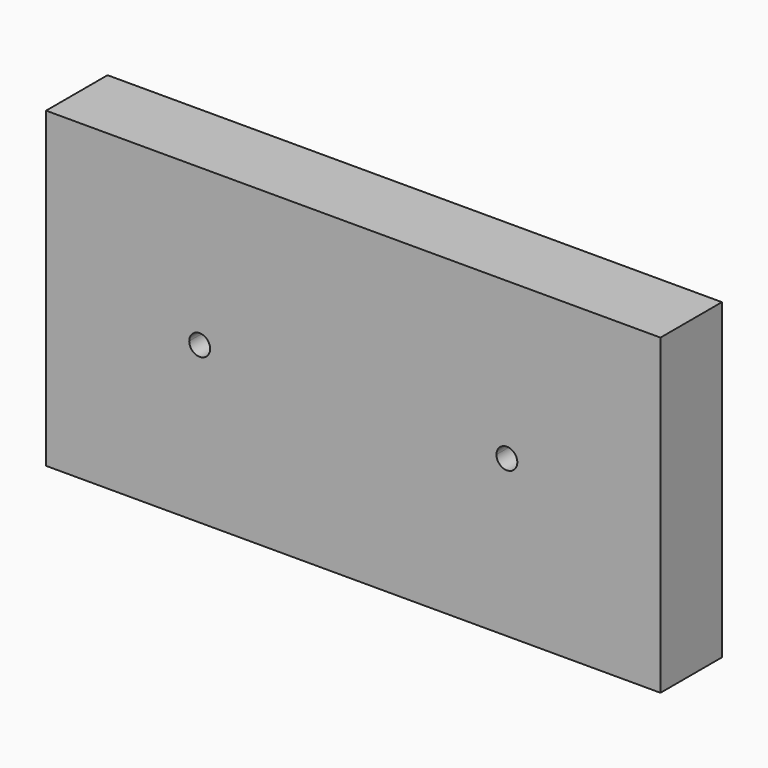
from build123d import *

# Parameters (mm, degrees)
F1_DEPTH = 3.175


with BuildPart() as f1:
    # F0 (on Front) → F1 (new body)
    with BuildSketch(Plane.XZ):
        with BuildLine():
            Line((-18.7849326355, 12.9286), (-25.1349326355, 12.9286))
            Line((-25.1349326355, 12.9286), (-25.1349326355, 6.4643))
            Line((-25.1349326355, 6.4643), (-19.2167326355, 6.4643))
            ThreePointArc((-19.2167326355, 6.4643), (-19.0902613436, 6.7696287081), (-18.7849326355, 6.8961))
            Line((-18.7849326355, 6.8961), (-18.7849326355, 12.9286))
        make_face()
        with BuildLine():
            Line((-12.4349326355, 12.9286), (-18.7849326355, 12.9286))
            Line((-18.7849326355, 12.9286), (-18.7849326355, 6.8961))
            ThreePointArc((-18.7849326355, 6.8961), (-18.4796039274, 6.7696287081), (-18.3531326355, 6.4643))
            Line((-18.3531326355, 6.4643), (-12.4349326355, 6.4643))
            Line((-12.4349326355, 6.4643), (-12.4349326355, 12.9286))
        make_face()
        with BuildLine():
            Line((-6.0849326355, 12.9286), (-12.4349326355, 12.9286))
            Line((-12.4349326355, 12.9286), (-12.4349326355, 6.4643))
            Line((-12.4349326355, 6.4643), (-6.5167326355, 6.4643))
            ThreePointArc((-6.5167326355, 6.4643), (-6.3902613436, 6.7696287081), (-6.0849326355, 6.8961))
            Line((-6.0849326355, 6.8961), (-6.0849326355, 12.9286))
        make_face()
        with BuildLine():
            Line((0.2650673645, 12.9286), (-6.0849326355, 12.9286))
            Line((-6.0849326355, 12.9286), (-6.0849326355, 6.8961))
            ThreePointArc((-6.0849326355, 6.8961), (-5.7796039274, 6.7696287081), (-5.6531326355, 6.4643))
            Line((-5.6531326355, 6.4643), (0.2650673645, 6.4643))
            Line((0.2650673645, 6.4643), (0.2650673645, 12.9286))
        make_face()
        with BuildLine():
            Line((-19.2167326355, 6.4643), (-25.1349326355, 6.4643))
            Line((-25.1349326355, 6.4643), (-25.1349326355, 0))
            Line((-25.1349326355, 0), (-12.4349326355, 0))
            Line((-12.4349326355, 0), (-12.4349326355, 6.4643))
            Line((-12.4349326355, 6.4643), (-18.3531326355, 6.4643))
            ThreePointArc((-18.3531326355, 6.4643), (-18.7849326355, 6.0325), (-19.2167326355, 6.4643))
        make_face()
        with BuildLine():
            Line((-6.5167326355, 6.4643), (-12.4349326355, 6.4643))
            Line((-12.4349326355, 6.4643), (-12.4349326355, 0))
            Line((-12.4349326355, 0), (0.2650673645, 0))
            Line((0.2650673645, 0), (0.2650673645, 6.4643))
            Line((0.2650673645, 6.4643), (-5.6531326355, 6.4643))
            ThreePointArc((-5.6531326355, 6.4643), (-6.0849326355, 6.0325), (-6.5167326355, 6.4643))
        make_face()
    extrude(amount=F1_DEPTH)


solid = f1.part
